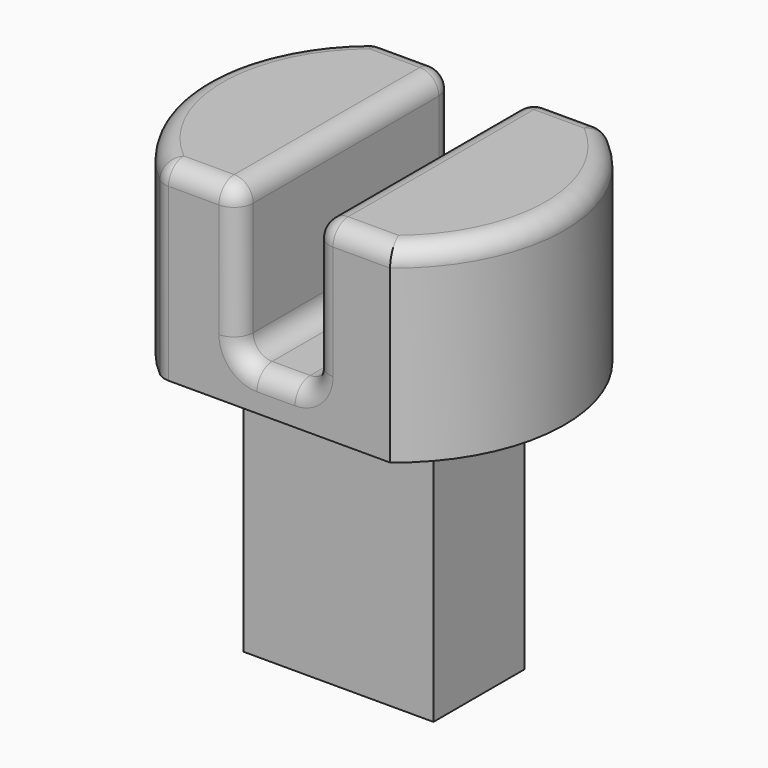
from build123d import *

# Parameters (mm, degrees)
F1_DEPTH = 5
F2_W     = 1
F2_H     = 7.1
F3_DEPTH = 4
F4_F1_R  = 0.5
F4_F2_R  = 0.5
F5_W     = 2.5
F5_H     = 1.5
F6_DEPTH = 7


with BuildPart() as f1:
    # F0 (on Top) → F1 (new body)
    with BuildSketch(Plane.XY):
        with BuildLine():
            Line((-6, 0), (-6, 7.1))
            ThreePointArc((-6, 7.1), (-7.75, 3.55), (-6, 0))
        make_face()
        Polygon((-3, 7.1), (-6, 7.1), (-6, 0), (-3, 0), (-3, 3.55), align=None)
        Polygon((0, 7.1), (-3, 7.1), (-3, 3.55), (-3, 0), (0, 0), align=None)
        with BuildLine():
            ThreePointArc((0, 0), (1.75, 3.55), (0, 7.1))
            Line((0, 7.1), (0, 0))
        make_face()
    extrude(amount=F1_DEPTH)

    # F2 (on face) → F3 (cut)
    with BuildSketch(Plane.XY.offset(5)):
        with Locations((-3.5, 3.55)):
            Rectangle(F2_W, F2_H)
        with Locations((-2.5, 3.55)):
            Rectangle(F2_W, F2_H)
    extrude(amount=-F3_DEPTH, mode=Mode.SUBTRACT)

    # F4: fillet of radius 0.5 on 15 edges, made by hand

    # F4_f1
    f4_f1_edges = [f1.edges().sort_by_distance(p)[0] for p in [
        (-4, 3.55, 1),
        (-2, 3.55, 1),
    ]]
    fillet(f4_f1_edges, radius=F4_F1_R)

    # F4_f2
    f4_f2_edges = [f1.edges().sort_by_distance(p)[0] for p in [
        (-5, 7.1, 5),
        (-4, 3.55, 5),
        (-5, 0, 5),
        (-7.75, 3.55, 5),
        (-1, 7.1, 5),
        (1.75, 3.55, 5),
        (-1, 0, 5),
        (-2, 3.55, 5),
        (-3, 0, 1),
        (-3, 7.1, 1),
        (0, 7.1, 2.5),
        (-6, 7.1, 2.5),
        (-6, 0, 2.5),
        (-2.1464466094, 7.1, 1.1464466094),
        (-3.8535533906, 7.1, 1.1464466094),
        (-3.8535533906, 0, 1.1464466094),
        (-2.1464466094, 0, 1.1464466094),
    ]]
    fillet(f4_f2_edges, radius=F4_F2_R)

    # F5 (on face) → F6 (join)
    with BuildSketch(Plane(origin=(0, 0, 0), x_dir=(1, 0, 0), z_dir=(0, 0, -1))):
        with Locations((-4.25, -2.8)):
            Rectangle(F5_W, F5_H)
        with Locations((-1.75, -2.8)):
            Rectangle(F5_W, F5_H)
        with Locations((-1.75, -4.3)):
            Rectangle(F5_W, F5_H)
        with Locations((-4.25, -4.3)):
            Rectangle(F5_W, F5_H)
    extrude(amount=F6_DEPTH)


solid = f1.part
